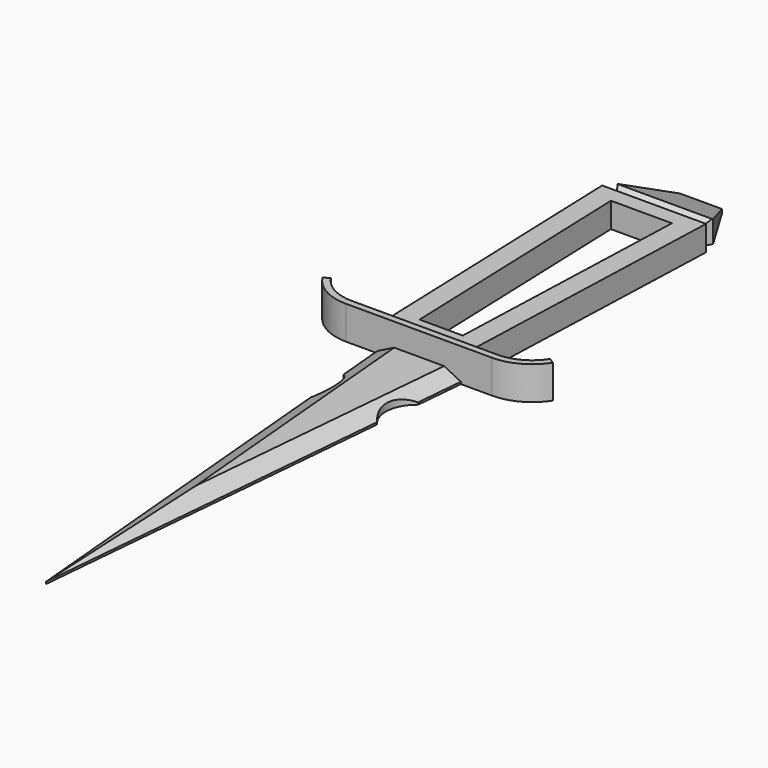
from build123d import *

# Parameters (mm, degrees)
F1_DEPTH     = 7.62
F2_W         = 26.67
F2_H         = 5.08
F3_DEPTH     = 0.508
F5_DEPTH     = 7.62
F7_DEPTH     = 25.4
F8_T1_DEPTH  = 39.5884897473
F8_T3_DEPTH  = 43.1891092466
F8_T5_DEPTH  = 15.7316119842
F8_T10_DEPTH = 21.2484768612
F8_T15_DEPTH = 21.2484768612
F8_T20_DEPTH = 21.2484768612
F8_T25_DEPTH = 21.2484768612
F10_DEPTH    = 10.16
F12_DEPTH    = 3.175
F13_C1_SIZE2 = 5.08
F13_C1_SIZE  = 2.54
F13_C2_SIZE2 = 2.54
F13_C2_SIZE  = 5.08


# Not quite as in the source:
# - a fillet or chamfer that OpenCascade refuses, or shapes differently, is made with other operations: its cross-section is extruded or revolved along the edge and cut away or added


with BuildPart() as f1:
    # F0 (on Top) → F1 (new body)
    with BuildSketch(Plane.XY):
        Polygon((-15.875, 88.9), (-12.7, 0), (12.7, 0), (15.875, 88.9), align=None)
        Polygon((-6.5727372599, 6.35), (-9.2941658314, 82.55), (9.2941658314, 82.55), (6.5727372599, 6.35), align=None, mode=Mode.SUBTRACT)
    extrude(amount=F1_DEPTH)

    # F2 (on face) → F3 (join)
    with BuildSketch(Plane(origin=(0, 88.9, 0), x_dir=(-1, 0, 0), z_dir=(0, 1, 0))):
        with Locations((0, 2.54)):
            Rectangle(F2_W, F2_H)
    extrude(amount=F3_DEPTH)

    # F4 (on Top) → F5 (join, through all)
    with BuildSketch(Plane.XY):
        Polygon((-6.35, 105.2430003945), (-15.875, 89.408), (15.875, 89.408), (6.35, 105.2430003945), align=None)
    extrude(amount=F5_DEPTH)

    # F6 (on Right) → F7 (cut, symmetric)
    with BuildSketch(Plane.YZ):
        Polygon((105.2430003945, 7.62), (89.408, 7.62), (105.2430003945, 1.27), align=None)
    extrude(amount=F7_DEPTH, both=True, mode=Mode.SUBTRACT)

    # F8: chamfer of 1.524 on 6 edges, made by hand

    # F8_s2 → F8_t1 (cut)
    with BuildSketch(Plane.YZ.offset(-19.7942448737)):
        Polygon((88.9, 6.096), (87.376, 7.62), (88.9, 7.62), align=None)
    extrude(amount=F8_T1_DEPTH, mode=Mode.SUBTRACT)

    # F8_s4 → F8_t3 (cut)
    with BuildSketch(Plane.YZ.offset(-21.5945546233)):
        Polygon((89.408, 5.3668893881), (91.4992312711, 6.7813944907), (89.408, 7.62), align=None)
    extrude(amount=F8_T3_DEPTH, mode=Mode.SUBTRACT)

    # F8_s6 → F8_t5 (cut)
    with BuildSketch(Plane.XY.offset(-4.0558059921)):
        Polygon((14.2955997995, 88.9), (15.8186287896, 87.3216061075), (15.875, 88.9), align=None)
        Polygon((-14.2955997995, 88.9), (-15.8186287896, 87.3216061075), (-15.875, 88.9), align=None)
    extrude(amount=F8_T5_DEPTH, mode=Mode.SUBTRACT)


with BuildPart() as f8_tool8:
    # F8_s9 → F8_t10 (new body)
    with BuildSketch(Plane.XY.offset(-6.8142384306)):
        Polygon((13.1798265815, 89.408), (14.4857717649, 91.7175464201), (15.875, 89.408), align=None)
    extrude(amount=F8_T10_DEPTH)

    split(bisect_by=Plane.YZ.offset(13.335), keep=Keep.TOP)


with BuildPart() as f1_1:
    add(f1.part)

    # F8_t7: cut F8_tool8
    add(f8_tool8.part, mode=Mode.SUBTRACT)


with BuildPart() as f8_tool13:
    # F8_s14 → F8_t15 (new body)
    with BuildSketch(Plane.XY.offset(-6.8142384306)):
        Polygon((13.1798265815, 89.408), (14.4857717649, 91.7175464201), (15.875, 89.408), align=None)
    extrude(amount=F8_T15_DEPTH)

    split(bisect_by=Plane.XY.offset(5.08), keep=Keep.TOP)


with BuildPart() as f1_2:
    add(f1_1.part)

    # F8_t12: cut F8_tool13
    add(f8_tool13.part, mode=Mode.SUBTRACT)


with BuildPart() as f8_tool18:
    # F8_s19 → F8_t20 (new body)
    with BuildSketch(Plane.XY.offset(-6.8142384306)):
        Polygon((-14.4857717649, 91.7175464201), (-13.1798265815, 89.408), (-15.875, 89.408), align=None)
    extrude(amount=F8_T20_DEPTH)

    split(bisect_by=Plane.YZ.offset(-13.335), keep=Keep.BOTTOM)


with BuildPart() as f1_3:
    add(f1_2.part)

    # F8_t17: cut F8_tool18
    add(f8_tool18.part, mode=Mode.SUBTRACT)


with BuildPart() as f8_tool23:
    # F8_s24 → F8_t25 (new body)
    with BuildSketch(Plane.XY.offset(-6.8142384306)):
        Polygon((-14.4857717649, 91.7175464201), (-13.1798265815, 89.408), (-15.875, 89.408), align=None)
    extrude(amount=F8_T25_DEPTH)

    split(bisect_by=Plane.XY.offset(5.08), keep=Keep.TOP)


with BuildPart() as f1_4:
    add(f1_3.part)

    # F8_t22: cut F8_tool23
    add(f8_tool23.part, mode=Mode.SUBTRACT)

    # F9 (on Top) → F10 (join)
    with BuildSketch(Plane.XY):
        with BuildLine():
            Line((22.2250049976, 0), (-22.2250049976, 0))
            ThreePointArc((-22.2250049976, 0), (-28.5750049976, 1.626602675), (-33.360963964, 6.1057692308))
            Line((-33.360963964, 6.1057692308), (-35.0741884204, 5.0131183432))
            ThreePointArc((-35.0741884204, 5.0131183432), (-29.5519258835, -0.155151961), (-22.225, -2.032))
            Line((-22.225, -2.032), (22.225, -2.032))
            ThreePointArc((22.225, -2.032), (29.5519258835, -0.155151961), (35.0741884204, 5.0131183432))
            Line((35.0741884204, 5.0131183432), (33.360963964, 6.1057692308))
            ThreePointArc((33.360963964, 6.1057692308), (28.5750049976, 1.626602675), (22.2250049976, 0))
        make_face()
    extrude(amount=F10_DEPTH)

    # F11 (on Top) → F12 (join)
    with BuildSketch(Plane.XY):
        with BuildLine():
            Line((12.7, -2.032), (-12.7, -2.032))
            Line((-12.7, -2.032), (-11.3907730168, -16.6665786134))
            ThreePointArc((-11.3907730168, -16.6665786134), (-7.6578884737, -23.408271606), (-10.1348339359, -30.7055034507))
            Line((-10.1348339359, -30.7055034507), (0, -143.9929821467))
            Line((0, -143.9929821467), (10.1348339359, -30.7055034507))
            ThreePointArc((10.1348339359, -30.7055034507), (7.6578884737, -23.408271606), (11.3907730168, -16.6665786134))
            Line((11.3907730168, -16.6665786134), (12.7, -2.032))
        make_face()
    extrude(amount=F12_DEPTH)

    # F13: chamfer of 2.54 x 5.08 on 4 edges, made by hand

    # F13_c1
    f13_c1_edges = [f1_4.edges().sort_by_distance(p)[0] for p in [
        (-12.0453865084, -9.3492893067, 3.175),
    ]]
    f13_c1_side = f1_4.faces().sort_by_distance((-12.0453865084, -9.3492893067, 3.1242))[0]
    chamfer(f13_c1_edges, length=F13_C1_SIZE, length2=F13_C1_SIZE2, reference=f13_c1_side)

    # F13_c2
    f13_c2_edges = [f1_4.edges().sort_by_distance(p)[0] for p in [
        (6.3424889397, -73.0964499313, 3.175),
    ]]
    f13_c2_side = f1_4.faces().sort_by_distance((6.2918910116, -73.0919233799, 3.175))[0]
    chamfer(f13_c2_edges, length=F13_C2_SIZE, length2=F13_C2_SIZE2, reference=f13_c2_side)


solid = f1_4.part
